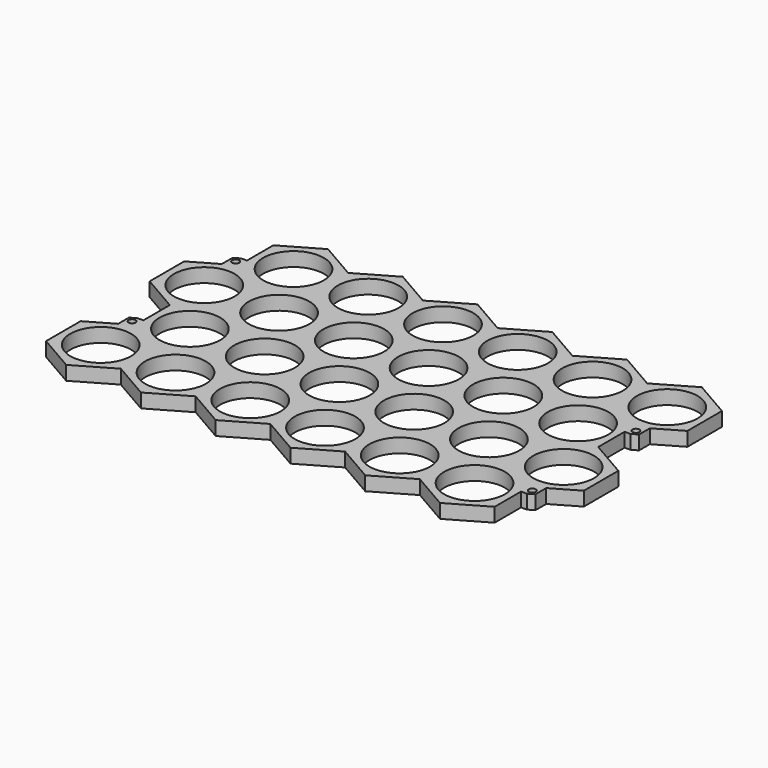
from build123d import *

# Parameters (mm, degrees)
F0_R     = 13
F0_R_2   = 1.5
F1_DEPTH = 6
F2_DEPTH = 6


# Not quite as in the source:
# - a feature names something its author has since deleted; it is built from what else it names


with BuildPart() as f1:
    # F0 (on Top) → F1 (new body)
    with BuildSketch(Plane.XY):
        Polygon((32, 18.4752086141), (16, 9.237604307), (16, -9.237604307), (32, -18.4752086141), (48, -9.237604307), (48, 9.237604307), align=None)
        with Locations((32, 0)):
            Circle(F0_R, mode=Mode.SUBTRACT)
        Polygon((16, -9.237604307), (16, 9.237604307), (0, 18.4752086141), (-2.5, 17.0318329411), (-5, 15.5884572681), (-16, 9.237604307), (-16, -9.237604307), (0, -18.4752086141), align=None)
        Circle(F0_R, mode=Mode.SUBTRACT)
        Polygon((0, 18.4752086141), (16, 9.237604307), (32, 18.4752086141), (32, 36.9504172281), (16, 46.1880215352), (0, 36.9504172281), (0, 22.805335633), (0, 21.36195996), align=None)
        with Locations((16, 27.7128129211)):
            Circle(F0_R, mode=Mode.SUBTRACT)
        Polygon((-2.5, 17.0318329411), (0, 18.4752086141), (0, 21.36195996), (-2.5, 22.805335633), (-5, 21.36195996), (-5, 18.4752086141), align=None)
        with Locations((-2.5, 19.918584287)):
            Circle(F0_R_2, mode=Mode.SUBTRACT)
        Polygon((32, 36.9504172281), (32, 18.4752086141), (48, 9.237604307), (64, 18.4752086141), (64, 36.9504172281), (48, 46.1880215352), align=None)
        with Locations((48, 27.7128129211)):
            Circle(F0_R, mode=Mode.SUBTRACT)
        Polygon((64, 18.4752086141), (48, 9.237604307), (48, -9.237604307), (64, -18.4752086141), (80, -9.237604307), (80, 9.237604307), align=None)
        with Locations((64, 0)):
            Circle(F0_R, mode=Mode.SUBTRACT)
        Polygon((16, 46.1880215352), (32, 36.9504172281), (48, 46.1880215352), (48, 64.6632301492), (32, 73.9008344563), (16, 64.6632301492), align=None)
        with Locations((32, 55.4256258422)):
            Circle(F0_R, mode=Mode.SUBTRACT)
        Polygon((64, 36.9504172281), (64, 18.4752086141), (80, 9.237604307), (96, 18.4752086141), (96, 36.9504172281), (80, 46.1880215352), align=None)
        with Locations((80, 27.7128129211)):
            Circle(F0_R, mode=Mode.SUBTRACT)
        Polygon((0, 36.9504172281), (16, 46.1880215352), (16, 64.6632301492), (0, 73.9008344563), (-2.5, 72.4574587833), (-5, 71.0140831103), (-16, 64.6632301492), (-16, 46.1880215352), align=None)
        with Locations((0, 55.4256258422)):
            Circle(F0_R, mode=Mode.SUBTRACT)
        Polygon((48, 64.6632301492), (48, 46.1880215352), (64, 36.9504172281), (80, 46.1880215352), (80, 64.6632301492), (64, 73.9008344563), align=None)
        with Locations((64, 55.4256258422)):
            Circle(F0_R, mode=Mode.SUBTRACT)
        Polygon((96, 18.4752086141), (80, 9.237604307), (80, -9.237604307), (96, -18.4752086141), (112, -9.237604307), (112, 9.237604307), align=None)
        with Locations((96, 0)):
            Circle(F0_R, mode=Mode.SUBTRACT)
        Polygon((32, 73.9008344563), (48, 64.6632301492), (64, 73.9008344563), (64, 92.3760430703), (48, 101.6136473774), (32, 92.3760430703), align=None)
        with Locations((48, 83.1384387633)):
            Circle(F0_R, mode=Mode.SUBTRACT)
        Polygon((96, 36.9504172281), (96, 18.4752086141), (112, 9.237604307), (128, 18.4752086141), (128, 36.9504172281), (112, 46.1880215352), align=None)
        with Locations((112, 27.7128129211)):
            Circle(F0_R, mode=Mode.SUBTRACT)
        Polygon((80, 64.6632301492), (80, 46.1880215352), (96, 36.9504172281), (112, 46.1880215352), (112, 64.6632301492), (96, 73.9008344563), align=None)
        with Locations((96, 55.4256258422)):
            Circle(F0_R, mode=Mode.SUBTRACT)
        Polygon((-2.5, 72.4574587833), (0, 73.9008344563), (0, 76.7875858022), (-2.5, 78.2309614752), (-5, 76.7875858022), (-5, 73.9008344563), align=None)
        with Locations((-2.5, 75.3442101292)):
            Circle(F0_R_2, mode=Mode.SUBTRACT)
        Polygon((64, 92.3760430703), (64, 73.9008344563), (80, 64.6632301492), (96, 73.9008344563), (96, 92.3760430703), (80, 101.6136473774), align=None)
        with Locations((80, 83.1384387633)):
            Circle(F0_R, mode=Mode.SUBTRACT)
        Polygon((128, 18.4752086141), (112, 9.237604307), (112, -9.237604307), (128, -18.4752086141), (144, -9.237604307), (144, 9.237604307), align=None)
        with Locations((128, 0)):
            Circle(F0_R, mode=Mode.SUBTRACT)
        Polygon((128, 36.9504172281), (128, 18.4752086141), (144, 9.237604307), (160, 18.4752086141), (160, 36.9504172281), (144, 46.1880215352), align=None)
        with Locations((144, 27.7128129211)):
            Circle(F0_R, mode=Mode.SUBTRACT)
        Polygon((112, 64.6632301492), (112, 46.1880215352), (128, 36.9504172281), (144, 46.1880215352), (144, 64.6632301492), (128, 73.9008344563), align=None)
        with Locations((128, 55.4256258422)):
            Circle(F0_R, mode=Mode.SUBTRACT)
        Polygon((96, 92.3760430703), (96, 73.9008344563), (112, 64.6632301492), (128, 73.9008344563), (128, 92.3760430703), (112, 101.6136473774), align=None)
        with Locations((112, 83.1384387633)):
            Circle(F0_R, mode=Mode.SUBTRACT)
        Polygon((160, 18.4752086141), (144, 9.237604307), (144, -9.237604307), (160, -18.4752086141), (176, -9.237604307), (176, 4.9074772881), (176, 6.3508529611), (176, 9.237604307), align=None)
        with Locations((160, 0)):
            Circle(F0_R, mode=Mode.SUBTRACT)
        Polygon((160, 36.9504172281), (160, 18.4752086141), (176, 9.237604307), (178.5, 10.68097998), (181, 12.124355653), (192, 18.4752086141), (192, 36.9504172281), (176, 46.1880215352), align=None)
        with Locations((176, 27.7128129211)):
            Circle(F0_R, mode=Mode.SUBTRACT)
        Polygon((144, 64.6632301492), (144, 46.1880215352), (160, 36.9504172281), (176, 46.1880215352), (176, 60.3331031303), (176, 61.7764788033), (176, 64.6632301492), (160, 73.9008344563), align=None)
        with Locations((160, 55.4256258422)):
            Circle(F0_R, mode=Mode.SUBTRACT)
        Polygon((128, 92.3760430703), (128, 73.9008344563), (144, 64.6632301492), (160, 73.9008344563), (160, 92.3760430703), (144, 101.6136473774), align=None)
        with Locations((144, 83.1384387633)):
            Circle(F0_R, mode=Mode.SUBTRACT)
        Polygon((160, 92.3760430703), (160, 73.9008344563), (176, 64.6632301492), (178.5, 66.1066058222), (181, 67.5499814952), (192, 73.9008344563), (192, 92.3760430703), (176, 101.6136473774), align=None)
        with Locations((176, 83.1384387633)):
            Circle(F0_R, mode=Mode.SUBTRACT)
    extrude(amount=F1_DEPTH)

    # F0 (on Top) → F2 (join)
    with BuildSketch(Plane.XY):
        Polygon((0, 18.4752086141), (16, 9.237604307), (32, 18.4752086141), (32, 36.9504172281), (16, 46.1880215352), (0, 36.9504172281), (0, 22.805335633), (0, 21.36195996), align=None)
        with Locations((16, 27.7128129211)):
            Circle(F0_R, mode=Mode.SUBTRACT)
        Polygon((0, 73.9008344563), (16, 64.6632301492), (32, 73.9008344563), (32, 92.3760430703), (16, 101.6136473774), (0, 92.3760430703), (0, 78.2309614752), (0, 76.7875858022), align=None)
        with Locations((16, 83.1384387633)):
            Circle(F0_R, mode=Mode.SUBTRACT)
        Polygon((178.5, 10.68097998), (176, 9.237604307), (176, 6.3508529611), (178.5, 4.9074772881), (181, 6.3508529611), (181, 9.237604307), align=None)
        with Locations((178.5, 7.7942286341)):
            Circle(F0_R_2, mode=Mode.SUBTRACT)
        Polygon((178.5, 66.1066058222), (176, 64.6632301492), (176, 61.7764788033), (178.5, 60.3331031303), (181, 61.7764788033), (181, 64.6632301492), align=None)
        with Locations((178.5, 63.2198544763)):
            Circle(F0_R_2, mode=Mode.SUBTRACT)
        Polygon((-5, 71.0140831103), (-2.5, 72.4574587833), (-5, 73.9008344563), align=None)
        Polygon((-2.5, 78.2309614752), (0, 76.7875858022), (0, 78.2309614752), align=None)
        Polygon((-2.5, 22.805335633), (0, 21.36195996), (0, 22.805335633), align=None)
        Polygon((-5, 15.5884572681), (-2.5, 17.0318329411), (-5, 18.4752086141), align=None)
        Polygon((176, 61.7764788033), (176, 60.3331031303), (178.5, 60.3331031303), align=None)
        Polygon((181, 67.5499814952), (178.5, 66.1066058222), (181, 64.6632301492), align=None)
        Polygon((178.5, 4.9074772881), (176, 6.3508529611), (176, 4.9074772881), align=None)
        Polygon((181, 12.124355653), (178.5, 10.68097998), (181, 9.237604307), align=None)
    extrude(amount=F2_DEPTH)


solid = f1.part
